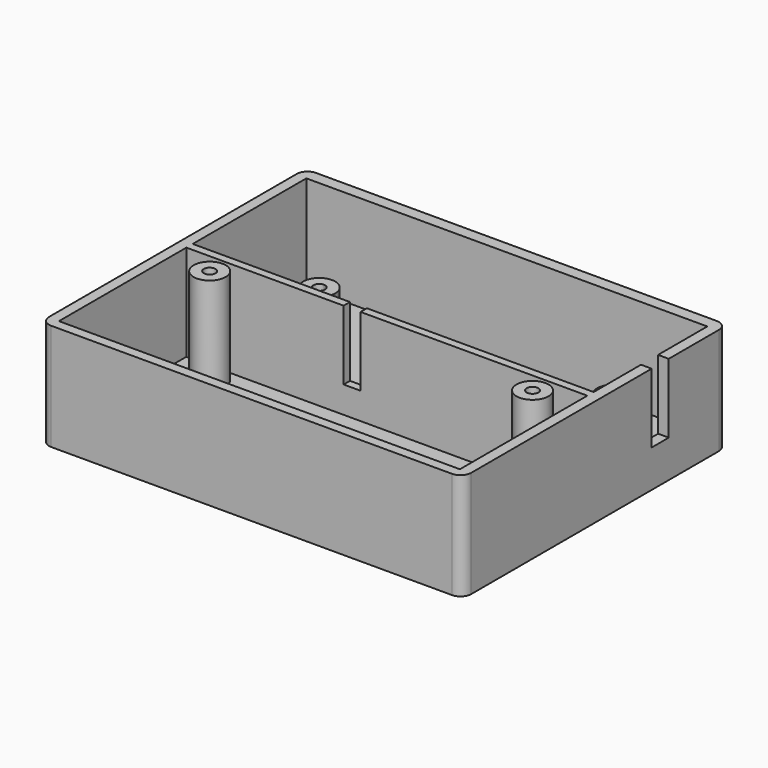
from build123d import *

# Parameters (mm, degrees)
F1_DEPTH = 20
F0_R     = 3
F0_R_2   = 1.1
F2_DEPTH = 2
F3_DEPTH = 10.75
F0_W     = 3.1642657705
F0_H     = 1.4890261218
F4_DEPTH = 7
F5_R     = 2


# Not quite as in the source:
# - a feature names something its author has since deleted; it is built from what else it names


with BuildPart() as f1:
    # F0 (on Top) → F1 (new body)
    with BuildSketch(Plane.XY):
        Polygon((-37.55, -13.0740804598), (-37.55, -12.1), (-37.55, 13.5259195402), (37.55, 13.5259195402), (37.55, 2.0000108369), (39.55, 2.0000108369), (39.55, 15.7519578086), (-39.5226512551, 15.7519578086), (-39.5226512551, -46.2480421914), (39.55, -46.2480421914), (39.55, -1.9999891631), (37.55, -1.9999891631), (37.55, -13.0740804598), (-4.9305087887, -13.0740804598), (-4.9305087887, -14.5631065816), (36.1, -14.5631065816), (37.55, -14.5631065816), (37.55, -44.3981406778), (-37.55, -44.3981406778), (-37.55, -14.5631065816), (-36.1, -14.5631065816), (-8.0947745591, -14.5631065816), (-8.0947745591, -13.0740804598), align=None)
    extrude(amount=F1_DEPTH)



with BuildPart() as f1b:
    # F0 (on Top) → F1, piece 2 (new body)
    with BuildSketch(Plane.XY):
        with Locations((-30.2370786667, -18.2506926358)):
            Circle(F0_R)
        with Locations((-30.2370786667, -18.2506926358)):
            Circle(F0_R_2, mode=Mode.SUBTRACT)
    extrude(amount=F1_DEPTH)


with BuildPart() as f1c:
    # F0 (on Top) → F1, piece 3 (new body)
    with BuildSketch(Plane.XY):
        with Locations((30.2370786667, -18.2506926358)):
            Circle(F0_R)
        with Locations((30.2370786667, -18.2506926358)):
            Circle(F0_R_2, mode=Mode.SUBTRACT)
    extrude(amount=F1_DEPTH)


with BuildPart() as f2:
    # F0 (on Top) → F2 (new body)
    with BuildSketch(Plane.XY):
        with BuildLine():
            Line((-25.6, 1.6), (-25.6, 2.7))
            ThreePointArc((-25.6, 2.7), (-26.3778174593, 0.8221825407), (-24.5, 1.6))
            Line((-24.5, 1.6), (-25.6, 1.6))
        make_face()
        with BuildLine():
            ThreePointArc((-24.5, 1.6), (-24.8221825407, 2.3778174593), (-25.6, 2.7))
            Line((-25.6, 2.7), (-25.6, 1.6))
            Line((-25.6, 1.6), (-24.5, 1.6))
        make_face()
    extrude(amount=F2_DEPTH)


with BuildPart() as f2b:
    # F0 (on Top) → F2, piece 2 (new body)
    with BuildSketch(Plane.XY):
        with BuildLine():
            ThreePointArc((30.2, 2.1), (29.8778174593, 2.8778174593), (29.1, 3.2))
            ThreePointArc((29.1, 3.2), (28.3221825407, 1.3221825407), (30.2, 2.1))
        make_face()
    extrude(amount=F2_DEPTH)


with BuildPart() as f1_1:
    add(f1.part)

    add(f1b.part)  # F2#3 merges F1b

    add(f1c.part)  # F2#3 merges F1c
    # F0 (on Top) → F2, piece 3 (join)
    with BuildSketch(Plane.XY):
        Polygon((-4.9305087887, -14.5631065816), (-8.0947745591, -14.5631065816), (-36.1, -14.5631065816), (-36.1, -42.9981406778), (36.1, -42.9981406778), (36.1, -14.5631065816), align=None)
        with Locations((-30.2370786667, -18.2506926358)):
            Circle(F0_R, mode=Mode.SUBTRACT)
        with Locations((30.2370786667, -18.2506926358)):
            Circle(F0_R, mode=Mode.SUBTRACT)
        Polygon((-37.55, 13.5259195402), (-37.55, -12.1), (-37.55, -13.0740804598), (-8.0947745591, -13.0740804598), (-4.9305087887, -13.0740804598), (37.55, -13.0740804598), (37.55, -1.9999891631), (37.55, 2.0000108369), (37.55, 13.5259195402), align=None)
        Polygon((36.1, 12.1), (36.1, -12.1), (-36.1, -12.1), (-36.1, 12.1), (-25.6, 12.1), (29.1, 12.1), align=None, mode=Mode.SUBTRACT)
        Polygon((-36.1, -12.1), (36.1, -12.1), (36.1, 12.1), (29.1, 12.1), (-25.6, 12.1), (-36.1, 12.1), align=None)
        with BuildLine():
            ThreePointArc((-22.6, 1.6), (-27.7213203436, -0.5213203436), (-25.6, 4.6))
            ThreePointArc((-25.6, 4.6), (-23.4786796564, 3.7213203436), (-22.6, 1.6))
        make_face(mode=Mode.SUBTRACT)
        with BuildLine():
            ThreePointArc((32.1000297599, 2.1), (26.978658613, -0.021341387), (29.1, 5.1000297599))
            ThreePointArc((29.1, 5.1000297599), (31.221341387, 4.221341387), (32.1000297599, 2.1))
        make_face(mode=Mode.SUBTRACT)
        Polygon((-36.1, -42.9981406778), (-36.1, -14.5631065816), (-37.55, -14.5631065816), (-37.55, -44.3981406778), (37.55, -44.3981406778), (37.55, -14.5631065816), (36.1, -14.5631065816), (36.1, -42.9981406778), align=None)
        with Locations((-30.2370786667, -18.2506926358)):
            Circle(F0_R_2)
        with Locations((30.2370786667, -18.2506926358)):
            Circle(F0_R_2)
    extrude(amount=F2_DEPTH)


    add(f2.part)  # F3 merges F2

    add(f2b.part)  # F3 merges F2b
    # F0 (on Top) → F3 (join)
    with BuildSketch(Plane.XY):
        with BuildLine():
            Line((-25.6, 2.7), (-25.6, 4.6))
            ThreePointArc((-25.6, 4.6), (-27.7213203436, -0.5213203436), (-22.6, 1.6))
            Line((-22.6, 1.6), (-24.5, 1.6))
            ThreePointArc((-24.5, 1.6), (-26.3778174593, 0.8221825407), (-25.6, 2.7))
        make_face()
        with BuildLine():
            ThreePointArc((-22.6, 1.6), (-23.4786796564, 3.7213203436), (-25.6, 4.6))
            Line((-25.6, 4.6), (-25.6, 2.7))
            ThreePointArc((-25.6, 2.7), (-24.8221825407, 2.3778174593), (-24.5, 1.6))
            Line((-24.5, 1.6), (-22.6, 1.6))
        make_face()
        with BuildLine():
            ThreePointArc((32.1000297599, 2.1), (31.221341387, 4.221341387), (29.1, 5.1000297599))
            ThreePointArc((29.1, 5.1000297599), (26.978658613, -0.021341387), (32.1000297599, 2.1))
        make_face()
        with BuildLine():
            ThreePointArc((30.2, 2.1), (28.3221825407, 1.3221825407), (29.1, 3.2))
            ThreePointArc((29.1, 3.2), (29.8778174593, 2.8778174593), (30.2, 2.1))
        make_face(mode=Mode.SUBTRACT)
    extrude(amount=F3_DEPTH)

    # F0 (on Top) → F4 (join)
    with BuildSketch(Plane.XY):
        Polygon((39.55, 2.0000108369), (37.55, 2.0000108369), (37.55, -1.9999891631), (39.55, -1.9999891631), (39.55, 1.08369e-05), align=None)
        with Locations((-6.5126416739, -13.8185935207)):
            Rectangle(F0_W, F0_H)
    extrude(amount=F4_DEPTH)

    # F5
    f5_edges = [f1_1.edges().sort_by_distance(p)[0] for p in [
        (39.55, -46.248042, 10),
        (39.55, 15.751958, 10),
        (-39.522651, 15.751958, 10),
        (-39.522651, -46.248042, 10),
    ]]
    fillet(f5_edges, radius=F5_R)


solid = f1_1.part
